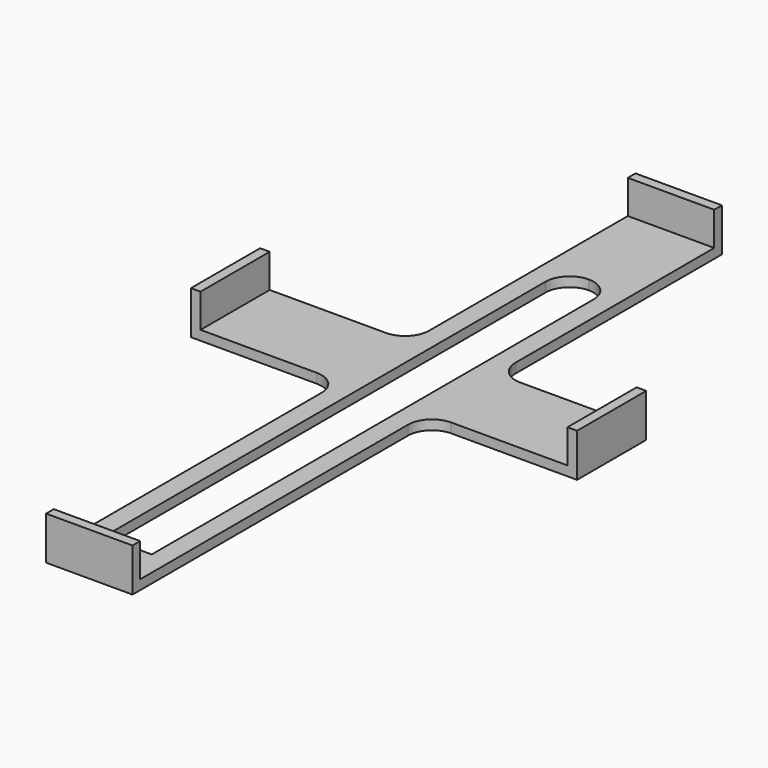
from build123d import *

# Parameters (mm, degrees)
F0_W     = 10
F0_H     = 120
F0_W_2   = 31.2
F0_H_2   = 18
F1_DEPTH = 2
F3_W     = 2
F3_H     = 18
F3_W_2   = 18
F3_H_2   = 2
F4_DEPTH = 7
F5_R     = 4.99999


# Not quite as in the source:
# - a fillet or chamfer is up to 0.001 mm smaller than in the source, because OpenCascade refuses the exact size


with BuildPart() as f1:
    # F0 (on Top) → F1 (new body)
    with BuildSketch(Plane.XY):
        Polygon((9, 135.3739356415), (-9, 135.3739356415), (-9, 76.6739356415), (-9, 58.6739356415), (-9, -18.0260643585), (9, -18.0260643585), (9, 58.6739356415), (9, 76.6739356415), align=None)
        with Locations((0, 51.9739356415)):
            Rectangle(F0_W, F0_H, mode=Mode.SUBTRACT)
        with Locations((-24.6, 67.6739356415)):
            Rectangle(F0_W_2, F0_H_2)
        with Locations((24.6, 67.6739356415)):
            Rectangle(F0_W_2, F0_H_2)
    extrude(amount=F1_DEPTH)

    # F3 (on face) → F4 (join)
    with BuildSketch(Plane.XY.offset(2)):
        with Locations((-39.2, 67.6739356415)):
            Rectangle(F3_W, F3_H)
        with Locations((39.2, 67.6739356415)):
            Rectangle(F3_W, F3_H)
        with Locations((0, 134.3739356415)):
            Rectangle(F3_W_2, F3_H_2)
        with Locations((0, -17.0260643585)):
            Rectangle(F3_W_2, F3_H_2)
    extrude(amount=F4_DEPTH)

    # F5 (radius 5 in the source; OpenCascade refuses exactly that, so slightly less here)
    f5_edges = [f1.edges().sort_by_distance(p)[0] for p in [
        (-9, 58.673936, 1),
        (9, 58.673936, 1),
        (9, 76.673936, 1),
        (-9, 76.673936, 1),
        (-5, 111.973936, 1),
        (5, 111.973936, 1),
    ]]
    fillet(f5_edges, radius=F5_R)


solid = f1.part
